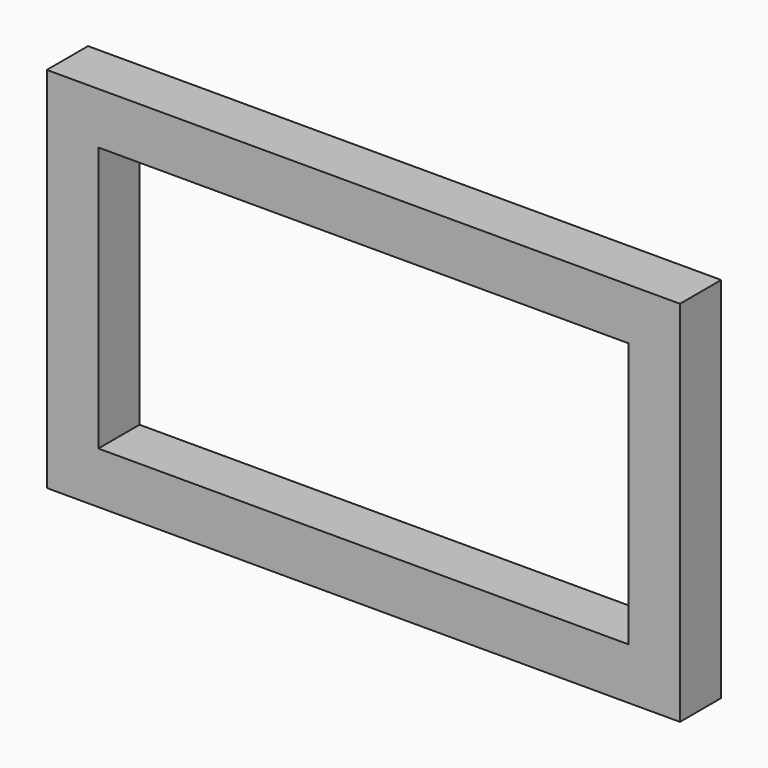
from build123d import *

# Parameters (mm, degrees)
F0_W          = 860
F0_H          = 500
F0_W_2        = 720
F0_H_2        = 360
F1_DEPTH      = 70
F3_W          = 30
F3_H          = 360
F4_DEPTH      = 25
F4_DEPTH_BACK = 25
F5_SCALE      = 0.4


# Not quite as in the source:
# - a feature names something its author has since deleted; it is built from what else it names


with BuildPart() as f1:
    # F0 (on Front) → F1 (new body)
    with BuildSketch(Plane.XZ):
        with Locations((-61.0144731402, -34.6215157021)):
            Rectangle(F0_W, F0_H)
        with Locations((-61.0144731402, -34.6215157021)):
            Rectangle(F0_W_2, F0_H_2, mode=Mode.SUBTRACT)
    extrude(amount=F1_DEPTH)

    # F3 (on face) → F4 (cut, two sides)
    with BuildSketch(Plane(origin=(-491.0144731402, 0, 0), x_dir=(0, -1, 0), z_dir=(-1, 0, 0))) as f4_sk:
        with Locations((35, -34.6215157021)):
            Rectangle(F3_W, F3_H)
    extrude(amount=F4_DEPTH, mode=Mode.SUBTRACT)
    extrude(f4_sk.sketch, amount=-F4_DEPTH_BACK, mode=Mode.SUBTRACT)


with BuildPart() as f1_1:
    # F5: moved
    add(f1.part.scale(F5_SCALE).moved(Location((-294.6086838841, 0, -170.7729094213))))


solid = f1_1.part
